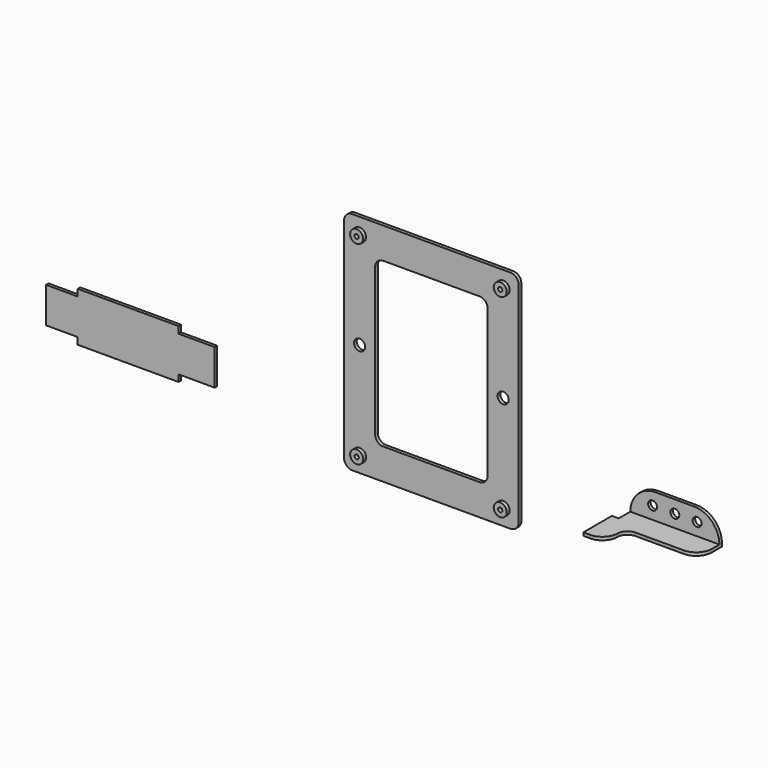
from build123d import *

# Parameters (mm, degrees)
F0_W      = 196.596
F0_H      = 254
F0_W_2    = 126.746
F0_H_2    = 184.15
F1_DEPTH  = 3.81
F2_R      = 9.2137253501
F3_R      = 6.2611
F4_DEPTH  = 3.81
F5_W      = 113.6904
F5_H      = 55.4228
F6_DEPTH  = 3.556
F7_W      = 100.33
F7_H      = 28.448
F8_DEPTH  = 3.556
F9_R      = 28.44799
F10_R     = 5.0165
F11_DEPTH = 3.556
F12_W     = 3.556
F12_H     = 40.1828
F13_DEPTH = 35.56
F14_W     = 3.556
F14_H     = 40.1828
F15_DEPTH = 40.64
F16_R     = 7.3025
F16_R_2   = 2.413
F17_DEPTH = 4.1402
F18_R     = 7.3025
F18_R_2   = 2.413
F19_DEPTH = 4.1402
F21_DEPTH = 3.556
F22_W     = 40.1828
F22_H     = 3.556
F23_DEPTH = 7.62
F24_R     = 17.6186891568


# Not quite as in the source:
# - a fillet or chamfer is up to 0.001 mm smaller than in the source, because OpenCascade refuses the exact size


with BuildPart() as f1:
    # F0 (on Front) → F1 (new body)
    with BuildSketch(Plane.XZ):
        with Locations((-7.8691132367, 30.2922270442)):
            Rectangle(F0_W, F0_H)
        with Locations((-7.8691132367, 30.2922270442)):
            Rectangle(F0_W_2, F0_H_2, mode=Mode.SUBTRACT)
    extrude(amount=F1_DEPTH)

    # F2
    f2_edges = [f1.edges().sort_by_distance(p)[0] for p in [
        (-106.167113, -1.905, 157.292227),
        (90.428887, -1.905, 157.292227),
        (90.428887, -1.905, -96.707773),
        (-106.167113, -1.905, -96.707773),
        (-71.242113, -1.905, -61.782773),
        (55.503887, -1.905, -61.782773),
        (55.503887, -1.905, 122.367227),
        (-71.242113, -1.905, 122.367227),
    ]]
    fillet(f2_edges, radius=F2_R)

    # F3 (on face) → F4 (cut, through all)
    with BuildSketch(Plane.XZ.offset(3.81)):
        with Locations((-88.7046132367, 30.2922270442)):
            Circle(F3_R)
        with Locations((72.9663867633, 30.2922270442)):
            Circle(F3_R)
    extrude(amount=-F4_DEPTH, mode=Mode.SUBTRACT)

    # F16 (on face) → F17 (join)
    with BuildSketch(Plane(origin=(0, 0, 0), x_dir=(-1, 0, 0), z_dir=(0, 1, 0))):
        with Locations((-72.9663867633, 139.5122270442)):
            Circle(F16_R)
        with Locations((-72.9663867633, 139.5122270442)):
            Circle(F16_R_2, mode=Mode.SUBTRACT)
        with Locations((88.7046132367, 139.5122270442)):
            Circle(F16_R)
        with Locations((88.7046132367, 139.5122270442)):
            Circle(F16_R_2, mode=Mode.SUBTRACT)
        with Locations((88.7046132367, -78.9277729558)):
            Circle(F16_R)
        with Locations((88.7046132367, -78.9277729558)):
            Circle(F16_R_2, mode=Mode.SUBTRACT)
        with Locations((-72.9663867633, -78.9277729558)):
            Circle(F16_R)
        with Locations((-72.9663867633, -78.9277729558)):
            Circle(F16_R_2, mode=Mode.SUBTRACT)
    extrude(amount=F17_DEPTH)

    # F18 (on face) → F19 (join)
    with BuildSketch(Plane.XZ.offset(3.81)):
        with Locations((72.9663867633, 139.5122270442)):
            Circle(F18_R)
        with Locations((72.9663867633, 139.5122270442)):
            Circle(F18_R_2, mode=Mode.SUBTRACT)
        with Locations((-88.7046132367, 139.5122270442)):
            Circle(F18_R)
        with Locations((-88.7046132367, 139.5122270442)):
            Circle(F18_R_2, mode=Mode.SUBTRACT)
        with Locations((-88.7046132367, -78.9277729558)):
            Circle(F18_R)
        with Locations((-88.7046132367, -78.9277729558)):
            Circle(F18_R_2, mode=Mode.SUBTRACT)
        with Locations((72.9663867633, -78.9277729558)):
            Circle(F18_R)
        with Locations((72.9663867633, -78.9277729558)):
            Circle(F18_R_2, mode=Mode.SUBTRACT)
    extrude(amount=F19_DEPTH)


with BuildPart() as f6:
    # F5 (on Front) → F6 (new body)
    with BuildSketch(Plane.XZ):
        with Locations((-349.5139063023, -45.2142719351)):
            Rectangle(F5_W, F5_H)
    extrude(amount=F6_DEPTH)

    # F12 (on face) → F13 (join)
    with BuildSketch(Plane(origin=(-406.3591063023, 0, 0), x_dir=(0, -1, 0), z_dir=(-1, 0, 0))):
        with Locations((1.778, -45.2142719351)):
            Rectangle(F12_W, F12_H)
    extrude(amount=F13_DEPTH)

    # F14 (on face) → F15 (join)
    with BuildSketch(Plane.YZ.offset(-292.6687063023)):
        with Locations((-1.778, -45.2142719351)):
            Rectangle(F14_W, F14_H)
    extrude(amount=F15_DEPTH)


with BuildPart() as f8:
    # F7 (on Front) → F8 (new body)
    with BuildSketch(Plane.XZ):
        with Locations((266.0880976948, -21.7766570859)):
            Rectangle(F7_W, F7_H)
    extrude(amount=F8_DEPTH)

    # F9 (radius 28.448 in the source; OpenCascade refuses exactly that, so slightly less here)
    f9_edges = [f8.edges().sort_by_distance(p)[0] for p in [
        (215.923098, -1.778, -7.552657),
        (316.253098, -1.778, -7.552657),
    ]]
    fillet(f9_edges, radius=F9_R)

    # F10 (on face) → F11 (cut, through all)
    with BuildSketch(Plane.XZ.offset(3.556)):
        with Locations((266.0880976948, -21.7766570859)):
            Circle(F10_R)
        with Locations((291.1705976948, -21.7766570859)):
            Circle(F10_R)
        with Locations((241.0055976948, -21.7766570859)):
            Circle(F10_R)
    extrude(amount=-F11_DEPTH, mode=Mode.SUBTRACT)


with BuildPart() as f21:
    # F20 (on face) → F21 (new body)
    with BuildSketch(Plane(origin=(0, 0, -36.0006570859), x_dir=(1, 0, 0), z_dir=(0, 0, -1))):
        with BuildLine():
            Line((215.9230976948, 0), (316.2530976948, 0))
            Line((316.2530976948, 0), (316.2530976948, 31.75))
            Line((316.2530976948, 31.75), (244.4805547121, 31.75))
            ThreePointArc((244.4805547121, 31.75), (236.1814756256, 35.3205988576), (233.0674678087, 43.8015684485))
            ThreePointArc((233.0674678087, 43.8015684485), (227.7561354432, 55.3854592004), (215.9230976948, 60.1157862604))
            Line((215.9230976948, 60.1157862604), (215.9230976948, 0))
        make_face()
    extrude(amount=F21_DEPTH)

    # F22 (on face) → F23 (join)
    with BuildSketch(Plane(origin=(215.9230976948, 0, 0), x_dir=(0, -1, 0), z_dir=(-1, 0, 0))):
        with Locations((40.0243862604, -37.7786570859)):
            Rectangle(F22_W, F22_H)
    extrude(amount=F23_DEPTH)

    # F24
    f24_edges = [f21.edges().sort_by_distance(p)[0] for p in [
        (316.253098, -31.75, -37.778657),
    ]]
    fillet(f24_edges, radius=F24_R)


solid = Compound([f1.part, f6.part, f8.part, f21.part])
